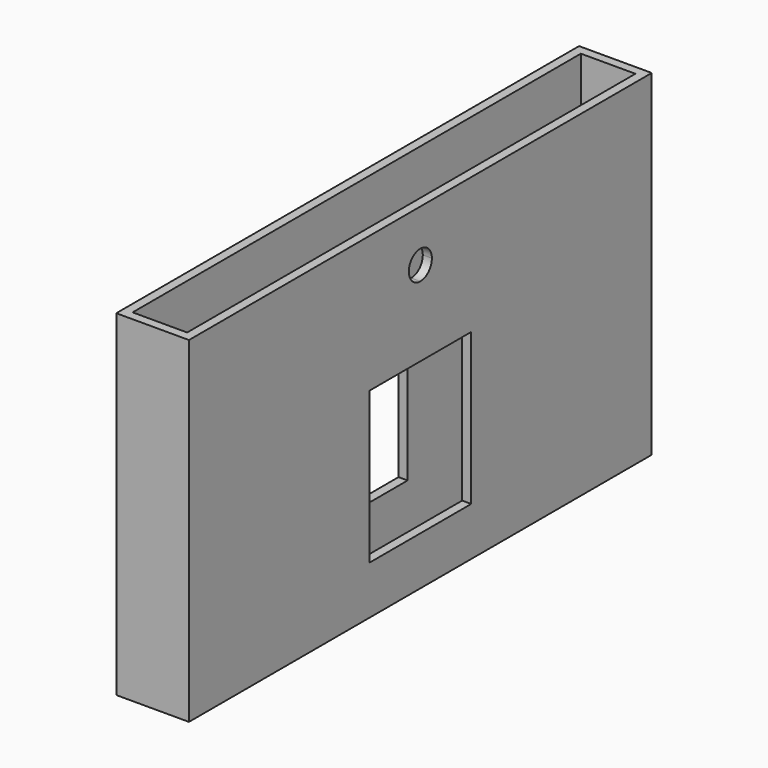
from build123d import *

# Parameters (mm, degrees)
F0_W     = 152.4
F0_H     = 1212.85
F0_W_2   = 114.3
F0_H_2   = 1174.75
F1_DEPTH = 704.85
F3_DEPTH = 25.4
F5_DEPTH = 19.05


# Not quite as in the source:
# - a feature names something its author has since deleted; it is built from what else it names


with BuildPart() as f1:
    # F0 (on Top) → F1 (new body)
    with BuildSketch(Plane.XY):
        Rectangle(F0_W, F0_H)
        Rectangle(F0_W_2, F0_H_2, mode=Mode.SUBTRACT)
    extrude(amount=F1_DEPTH)

    # F2 (on face) → F3 (cut)
    with BuildSketch(Plane.YZ.offset(76.2)):
        with BuildLine():
            ThreePointArc((30.226, 596.9), (-21.3730095681, 618.2730095681), (0, 566.674))
            ThreePointArc((0, 566.674), (21.3730095681, 575.5269904319), (30.226, 596.9))
        make_face()
        Polygon((-133.35, 101.6), (0, 101.6), (133.35, 101.6), (133.35, 419.1), (0, 419.1), (-133.35, 419.1), align=None)
    extrude(amount=-F3_DEPTH, mode=Mode.SUBTRACT)

    # F4 (on face) → F5 (cut)
    with BuildSketch(Plane(origin=(-76.2, 0, 0), x_dir=(0, -1, 0), z_dir=(-1, 0, 0))):
        Polygon((-133.35, 101.6), (0, 101.6), (133.35, 101.6), (133.35, 419.1), (-133.35, 419.1), align=None)
    extrude(amount=-F5_DEPTH, mode=Mode.SUBTRACT)


solid = f1.part
